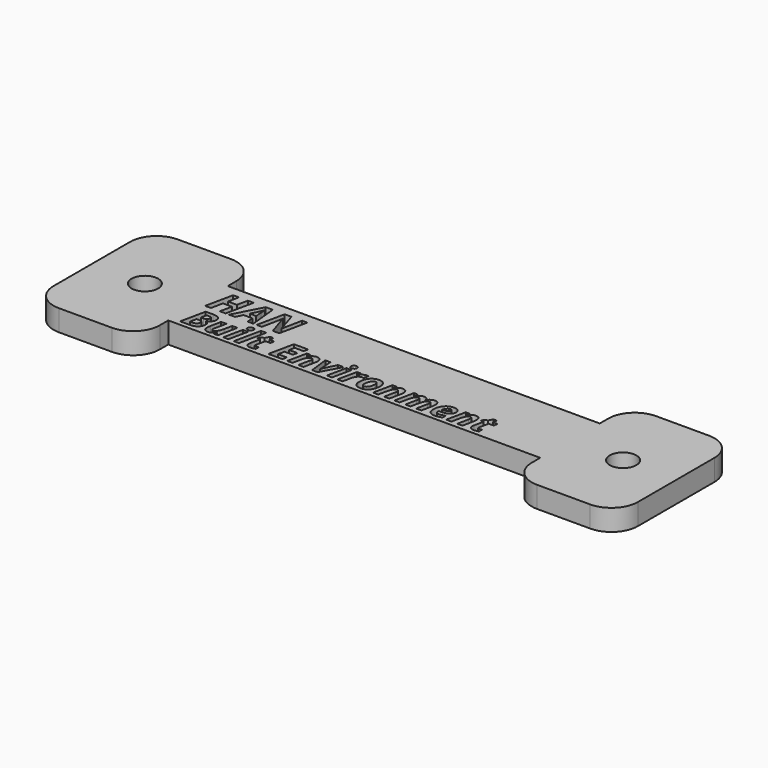
from build123d import *

# Parameters (mm, degrees)
F0_R         = 2.5
F1_DEPTH     = 4
F2_TEXT_SIZE = 7.3038041592
F3_DEPTH     = 5
F4_TEXT_SIZE = 6.6700600049
F5_DEPTH     = 5


# Not quite as in the source:
# - Text() gives the source's letters only with a copy of the font that has no kerning and outlines rounded to 1/6400 em; it was checked with that copy


with BuildPart() as f1:
    # F0 (on Top) → F1 (new body)
    with BuildSketch(Plane.XY):
        with BuildLine():
            Line((-55, 9), (-55, 0))
            Line((-55, 0), (-55, -9))
            ThreePointArc((-55, -9), (-53.5355339059, -12.5355339059), (-50, -14))
            Line((-50, -14), (-40, -14))
            ThreePointArc((-40, -14), (-36.4644660941, -12.5355339059), (-35, -9))
            Line((-35, -9), (-35, -7))
            Line((-35, -7), (35, -7))
            Line((35, -7), (35, -9))
            ThreePointArc((35, -9), (36.4644660941, -12.5355339059), (40, -14))
            Line((40, -14), (50, -14))
            ThreePointArc((50, -14), (53.5355339059, -12.5355339059), (55, -9))
            Line((55, -9), (55, 9))
            ThreePointArc((55, 9), (53.5355339059, 12.5355339059), (50, 14))
            Line((50, 14), (40, 14))
            ThreePointArc((40, 14), (36.4644660941, 12.5355339059), (35, 9))
            Line((35, 9), (35, 7))
            Line((35, 7), (-35, 7))
            Line((-35, 7), (-35, 9))
            ThreePointArc((-35, 9), (-36.4644660941, 12.5355339059), (-40, 14))
            Line((-40, 14), (-50, 14))
            ThreePointArc((-50, 14), (-53.5355339059, 12.5355339059), (-55, 9))
        make_face()
        with Locations((-45, 0)):
            Circle(F0_R, mode=Mode.SUBTRACT)
        with Locations((45, 0)):
            Circle(F0_R, mode=Mode.SUBTRACT)
    extrude(amount=-F1_DEPTH)

    # F2 (on Top) → F3 (cut)
    with BuildSketch(Plane.XY):
        with Locations((-33.8550843298, 0)):
            Text('HAN', F2_TEXT_SIZE, font='Open Sans', font_style=FontStyle.BOLDITALIC, text_align=(TextAlign.LEFT, TextAlign.BOTTOM))
    extrude(amount=-F3_DEPTH, mode=Mode.SUBTRACT)

    # F4 (on Top) → F5 (cut)
    with BuildSketch(Plane.XY):
        with Locations((-33.6220674217, -6.1454586685)):
            Text('Built Environment', F4_TEXT_SIZE, font='Open Sans', font_style=FontStyle.BOLDITALIC, text_align=(TextAlign.LEFT, TextAlign.BOTTOM))
    extrude(amount=-F5_DEPTH, mode=Mode.SUBTRACT)


solid = f1.part
